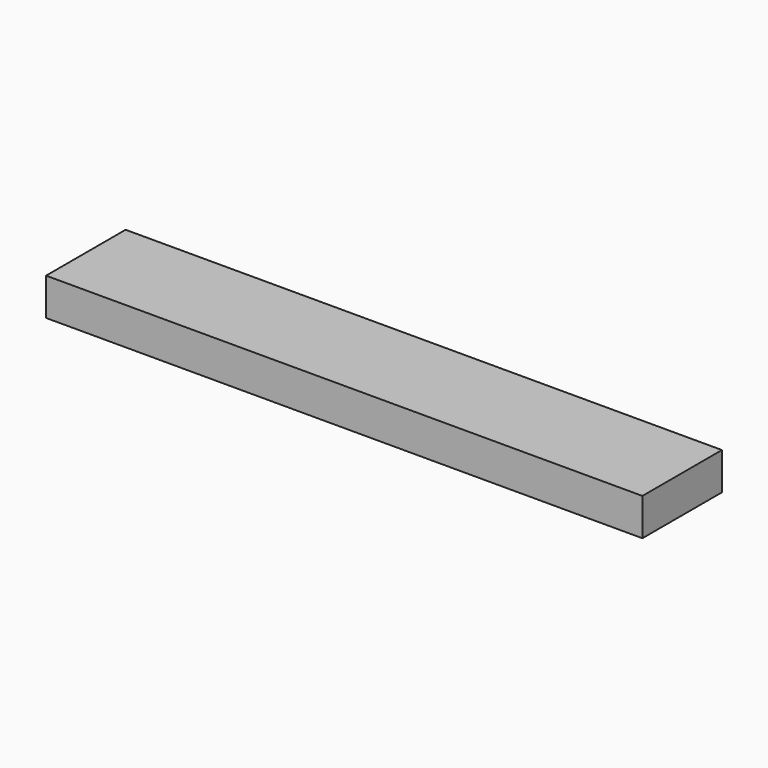
from build123d import *

# Parameters (mm, degrees)
F0_W     = 152.4
F0_H     = 25.4
F1_DEPTH = 9.525


# Not quite as in the source:
# - the program builds the solid bodies; features that only make, move or delete a surface that nothing else refers to are left out


with BuildPart() as f1:
    # F0 (on Top) → F1 (new body)
    with BuildSketch(Plane.XY):
        with Locations((76.2, 12.7)):
            Rectangle(F0_W, F0_H)
    extrude(amount=F1_DEPTH)


solid = f1.part
